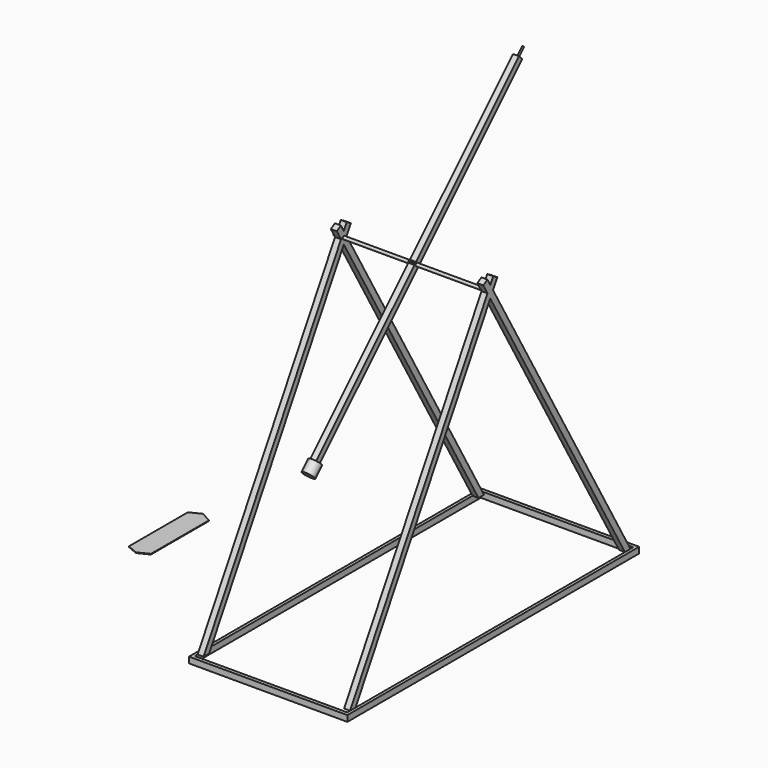
from build123d import *

# Parameters (mm, degrees)
F0_W         = 265
F0_H         = 610
F1_DEPTH     = 10
F2_W         = 255
F2_H         = 598
F3_DEPTH     = 25
F5_DEPTH     = 10
F8_R         = 2.5
F9_DEPTH     = 260
F10_W        = 10
F10_H        = 10
F11_DEPTH    = 520
F12_T1_DEPTH = 87.150489639
F13_W        = 10
F13_H        = 10
F14_DEPTH    = 305
F15_W        = 10
F15_H        = 478.3019721508
F16_DEPTH    = 25
F18_DEPTH    = 25
F20_DEPTH    = 25
F22_R        = 10
F23_DEPTH    = 10
F21_R        = 1.25
F24_DEPTH    = 15
F26_DEPTH    = 1


# Not quite as in the source:
# - a fillet or chamfer that OpenCascade refuses, or shapes differently, is made with other operations: its cross-section is extruded or revolved along the edge and cut away or added


with BuildPart() as f1:
    # F0 (on Top) → F1 (new body)
    with BuildSketch(Plane.XY):
        Rectangle(F0_W, F0_H)
    extrude(amount=F1_DEPTH)

    # F2 (on face) → F3 (cut)
    with BuildSketch(Plane.XY.offset(10)):
        Rectangle(F2_W, F2_H)
    extrude(amount=-F3_DEPTH, mode=Mode.SUBTRACT)


with BuildPart() as f5:
    # F4 (on face) → F5 (new body)
    with BuildSketch(Plane.YZ.offset(-127.5)):
        Polygon((6, 528.2754963085), (-293.2264973081, 10), (-281.6794919243, 10), (14.6602540378, 523.2754963085), align=None)
    extrude(amount=F5_DEPTH)


with BuildPart() as f6_1:
    # F6: instance of F5
    add(f5.part.mirror(Plane.YZ))


with BuildPart() as f7_1:
    # F7: instance of F5
    add(f5.part.mirror(Plane.XZ))


with BuildPart() as f7_2:
    # F7: instance of F6_1
    add(f6_1.part.mirror(Plane.XZ))


with BuildPart() as f5_1:
    add(f5.part)

    add(f6_1.part)  # F9 merges F6_1

    add(f7_1.part)  # F9 merges F7_1

    add(f7_2.part)  # F9 merges F7_2
    # F8 (on face) → F9 (join)
    with BuildSketch(Plane.YZ.offset(127.5)):
        with Locations((0, 508.0155730247)):
            Circle(F8_R)
    extrude(amount=-F9_DEPTH)


with BuildPart() as f11:
    # F10 (on Top) → F11 (new body)
    with BuildSketch(Plane.XY):
        with Locations((-0.6940327585, 0.4071239119)):
            Rectangle(F10_W, F10_H)
    extrude(amount=F11_DEPTH)

    # F12: chamfer of 15 on 1 edges, made by hand

    # F12_s2 → F12_t1 (cut)
    with BuildSketch(Plane.YZ.offset(-44.269277578)):
        Polygon((5.4071239119, 505), (-9.5928760881, 520), (5.4071239119, 520), align=None)
    extrude(amount=F12_T1_DEPTH, mode=Mode.SUBTRACT)

    # F15 (on face) → F16 (cut)
    with BuildSketch(Plane.YZ.offset(4.3059672415)):
        with Locations((0.4071239119, 239.1509860754)):
            Rectangle(F15_W, F15_H)
    extrude(amount=-F16_DEPTH, mode=Mode.SUBTRACT)

    # F17 (on face) → F18 (cut)
    with BuildSketch(Plane.YZ.offset(4.3059672415)):
        Polygon((5.4071239119, 478.3019721508), (5.4071239119, 505), (-4.5928760881, 495), (-4.5928760881, 478.3019721508), align=None)
    extrude(amount=-F18_DEPTH, mode=Mode.SUBTRACT)

    # F19 (on face) → F20 (cut)
    with BuildSketch(Plane.YZ.offset(4.3059672415)):
        Polygon((3.574793685, 520), (-4.5928760881, 520), (-4.5928760881, 511.8337869644), align=None)
    extrude(amount=-F20_DEPTH, mode=Mode.SUBTRACT)


with BuildPart() as f14:
    # F13 (on face) → F14 (new body, symmetric)
    with BuildSketch(Plane(origin=(0, 255.2035619559, 255.2035619559), x_dir=(-1, 0, 0), z_dir=(0, 0.7071067812, 0.7071067812))):
        with Locations((0.6940327585, 358.2655105144)):
            Rectangle(F13_W, F13_H)
    extrude(amount=F14_DEPTH, both=True)

    # F22 (on face) → F23 (join, symmetric)
    with BuildSketch(Plane(origin=(0, 39.535993694, 39.535993694), x_dir=(1, 0, 0), z_dir=(0, -0.7071067812, -0.7071067812))):
        with Locations((0, 358.2655105144)):
            Circle(F22_R)
    extrude(amount=F23_DEPTH, both=True)

    # F21 (on face) → F24 (join)
    with BuildSketch(Plane(origin=(0, 470.8711302178, 470.8711302178), x_dir=(-1, 0, 0), z_dir=(0, 0.7071067812, 0.7071067812))):
        with Locations((0, 358.2655105144)):
            Circle(F21_R)
    extrude(amount=F24_DEPTH)


with BuildPart() as f26:
    # F25 (on Top) → F26 (new body)
    with BuildSketch(Plane.XY):
        Polygon((-399.5258836659, 26.3972045484), (-399.5258836659, 20.4128491475), (-399.5258836659, -89.8914735812), (-399.5258836659, -96.8788117204), (-381.6058932129, -104.4853963744), (-363.7048708642, -95.5293477292), (-363.7048708642, -90.8532628168), (-363.7048708642, 17.6992724711), (-363.7238389685, 26.2021424537), (-381.6248613172, 35.3532531936), align=None)
    extrude(amount=F26_DEPTH)


solid = Compound([f1.part, f5_1.part, f11.part, f14.part, f26.part])
